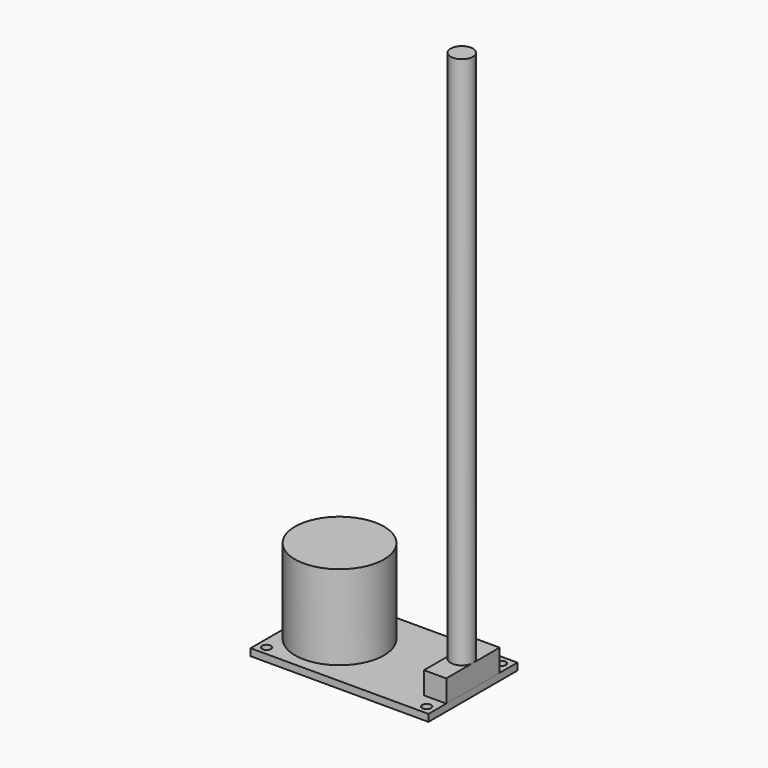
from build123d import *

# Parameters (mm, degrees)
F0_W     = 40
F0_H     = 25
F0_R     = 1
F1_DEPTH = 1.5875
F2_R     = 10
F3_DEPTH = 19
F4_W     = 5
F4_H     = 15
F5_DEPTH = 5
F6_R     = 2.5
F7_DEPTH = 120


# Not quite as in the source:
# - a length typed as a fraction of an inch, garbled in the dataset ("3 / 203.2 mm" for 3/8 in), is restored


with BuildPart() as f1:
    # F0 (on Top) → F1 (new body)
    with BuildSketch(Plane.XY):
        Rectangle(F0_W, F0_H)
        with Locations((-18, -10.5)):
            Circle(F0_R, mode=Mode.SUBTRACT)
        with Locations((18, -10.5)):
            Circle(F0_R, mode=Mode.SUBTRACT)
        with Locations((-18, 10.5)):
            Circle(F0_R, mode=Mode.SUBTRACT)
        with Locations((18, 10.5)):
            Circle(F0_R, mode=Mode.SUBTRACT)
    extrude(amount=F1_DEPTH)


with BuildPart() as f3:
    # F2 (on face) → F3 (new body)
    with BuildSketch(Plane.XY.offset(1.5875)):
        with Locations((-10, 0)):
            Circle(F2_R)
    extrude(amount=F3_DEPTH)


with BuildPart() as f5:
    # F4 (on face) → F5 (new body)
    with BuildSketch(Plane.XY.offset(1.5875)):
        with Locations((17.5, 0)):
            Rectangle(F4_W, F4_H)
    extrude(amount=F5_DEPTH)

    # F6 (on face) → F7 (join)
    with BuildSketch(Plane.XY.offset(6.5875)):
        with Locations((17.5, 0)):
            Circle(F6_R)
    extrude(amount=F7_DEPTH)


solid = Compound([f1.part, f3.part, f5.part])
